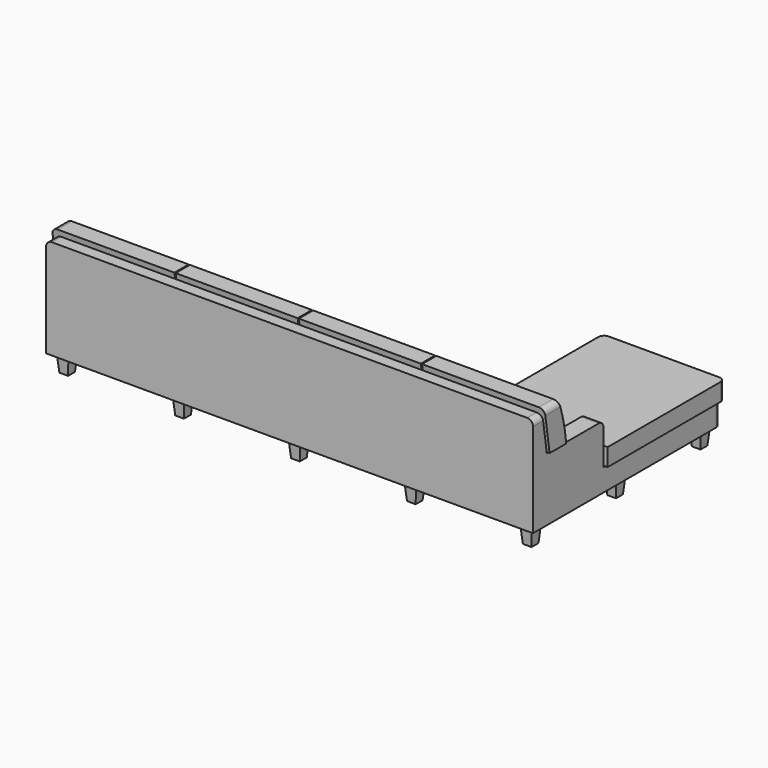
from build123d import *

# Parameters (mm, degrees)
F1_DEPTH       = 4150
F2_W           = 1000
F2_H           = 1100
F3_DEPTH       = 190
F4_W           = 150
F4_H           = 350
F5_DEPTH       = 750
F6_W           = 150
F6_H           = 540
F7_DEPTH       = 750
F9_DEPTH       = 150
F11_DEPTH      = 4175
F11_DEPTH_BACK = 25
F12_W          = 185
F12_H          = 210
F13_DEPTH      = 2020.001
F14_W          = 10
F14_H          = 920
F15_DEPTH      = 560.001
F15_DEPTH_BACK = 340.001
F16_R          = 50
F16_2_R        = 50
F16_3_R        = 50
F17_W          = 100
F17_H          = 100
F18_DEPTH      = 150
F18_TAPER      = 5


with BuildPart() as f1:
    # F0 (on Right) → F1 (new body)
    with BuildSketch(Plane.YZ):
        Polygon((0, 1000), (0, 150), (900, 150), (900, 340), (200, 340), (100, 1000), align=None)
    extrude(amount=F1_DEPTH)

    # F2 (on face) → F3 (join, through all)
    with BuildSketch(Plane(origin=(0, 0, 150), x_dir=(1, 0, 0), z_dir=(0, 0, -1))):
        with Locations((3650, -1450)):
            Rectangle(F2_W, F2_H)
    extrude(amount=-F3_DEPTH)

    # F4 (on Front) → F5 (join)
    with BuildSketch(Plane.XZ):
        with Locations((75, 515)):
            Rectangle(F4_W, F4_H)
    extrude(amount=-F5_DEPTH)

    # F6 (on Front) → F7 (join)
    with BuildSketch(Plane.XZ):
        with Locations((4075, 420)):
            Rectangle(F6_W, F6_H)
    extrude(amount=-F7_DEPTH)

    # F16
    f16_edges = [f1.edges().sort_by_distance(p)[0] for p in [
        (4150, 50, 1000),
        (4075, 750, 690),
        (4150, 2000, 245),
        (3150, 2000, 245),
        (0, 900, 245),
        (75, 750, 690),
        (0, 50, 1000),
    ]]
    fillet(f16_edges, radius=F16_R)


with BuildPart() as f9:
    # F8 (on face) → F9 (new body)
    with BuildSketch(Plane.XY.offset(340)):
        Polygon((3980, 770), (4170, 770), (4170, 2020), (3130, 2020), (3130, 920), (-20, 920), (-20, 770), (170, 770), (170, 220), (3980, 220), align=None)
    extrude(amount=F9_DEPTH)


with BuildPart() as f11:
    # F10 (on Right) → F11 (new body, two sides)
    with BuildSketch(Plane.YZ) as f11_sk:
        with BuildLine():
            Line((244.1362357722, 1050), (92.4242424242, 1050))
            Line((92.4242424242, 1050), (177.2727272727, 490))
            Line((177.2727272727, 490), (328.9847206207, 490))
            ThreePointArc((328.9847206207, 490), (313.2319068561, 774.0411255545), (244.1362357722, 1050))
        make_face()
    extrude(amount=F11_DEPTH)
    extrude(f11_sk.sketch, amount=-F11_DEPTH_BACK)

    # F12 (on Front) → F13 (cut, through all)
    with BuildSketch(Plane.XZ):
        with Locations((4082.5, 595)):
            Rectangle(F12_W, F12_H)
        with Locations((67.5, 595)):
            Rectangle(F12_W, F12_H)
    extrude(amount=-F13_DEPTH, mode=Mode.SUBTRACT)


with BuildPart() as f15_tool:
    # F14 (on face) → F15 (new body, two sides)
    with BuildSketch(Plane.XY.offset(490)) as f15_sk:
        with Locations((3125, 460)):
            Rectangle(F14_W, F14_H)
        with Locations((2075, 460)):
            Rectangle(F14_W, F14_H)
        with Locations((1025, 460)):
            Rectangle(F14_W, F14_H)
    extrude(amount=F15_DEPTH)
    extrude(f15_sk.sketch, amount=-F15_DEPTH_BACK)


with BuildPart() as f9_1:
    add(f9.part)

    # F15: cut by f15_tool
    add(f15_tool.part, mode=Mode.SUBTRACT)

    # F16#2
    f16_2_edges = [f9_1.edges().sort_by_distance(p)[0] for p in [
        (3130, 2020, 415),
        (4170, 2020, 415),
        (-20, 920, 415),
    ]]
    fillet(f16_2_edges, radius=F16_2_R)


with BuildPart() as f11_1:
    add(f11.part)

    # F15: cut by f15_tool
    add(f15_tool.part, mode=Mode.SUBTRACT)

    # F16#3
    f16_3_edges = [f11_1.edges().sort_by_distance(p)[0] for p in [
        (4175, 168.280239, 1050),
        (-25, 168.280239, 1050),
    ]]
    fillet(f16_3_edges, radius=F16_3_R)


with BuildPart() as f18:
    # F17 (on face) → F18 (new body, through all)
    with BuildSketch(Plane(origin=(0, 0, 150), x_dir=(1, 0, 0), z_dir=(0, 0, -1))):
        with Locations((100, -100)):
            Rectangle(F17_W, F17_H)
    extrude(amount=F18_DEPTH, taper=F18_TAPER)


with BuildPart() as f18b:
    # F17 (on face) → F18, piece 2 (new body, through all)
    with BuildSketch(Plane(origin=(0, 0, 150), x_dir=(1, 0, 0), z_dir=(0, 0, -1))):
        with Locations((1087.5, -100)):
            Rectangle(F17_W, F17_H)
    extrude(amount=F18_DEPTH, taper=F18_TAPER)


with BuildPart() as f18c:
    # F17 (on face) → F18, piece 3 (new body, through all)
    with BuildSketch(Plane(origin=(0, 0, 150), x_dir=(1, 0, 0), z_dir=(0, 0, -1))):
        with Locations((2075, -100)):
            Rectangle(F17_W, F17_H)
    extrude(amount=F18_DEPTH, taper=F18_TAPER)


with BuildPart() as f18d:
    # F17 (on face) → F18, piece 4 (new body, through all)
    with BuildSketch(Plane(origin=(0, 0, 150), x_dir=(1, 0, 0), z_dir=(0, 0, -1))):
        with Locations((100, -800)):
            Rectangle(F17_W, F17_H)
    extrude(amount=F18_DEPTH, taper=F18_TAPER)


with BuildPart() as f18e:
    # F17 (on face) → F18, piece 5 (new body, through all)
    with BuildSketch(Plane(origin=(0, 0, 150), x_dir=(1, 0, 0), z_dir=(0, 0, -1))):
        with Locations((1150, -800)):
            Rectangle(F17_W, F17_H)
    extrude(amount=F18_DEPTH, taper=F18_TAPER)


with BuildPart() as f18f:
    # F17 (on face) → F18, piece 6 (new body, through all)
    with BuildSketch(Plane(origin=(0, 0, 150), x_dir=(1, 0, 0), z_dir=(0, 0, -1))):
        with Locations((2200, -800)):
            Rectangle(F17_W, F17_H)
    extrude(amount=F18_DEPTH, taper=F18_TAPER)


with BuildPart() as f18g:
    # F17 (on face) → F18, piece 7 (new body, through all)
    with BuildSketch(Plane(origin=(0, 0, 150), x_dir=(1, 0, 0), z_dir=(0, 0, -1))):
        Polygon((4000, -1850), (4000, -1900), (4000, -1950), (4100, -1950), (4100, -1850), align=None)
    extrude(amount=F18_DEPTH, taper=F18_TAPER)


with BuildPart() as f18h:
    # F17 (on face) → F18, piece 8 (new body, through all)
    with BuildSketch(Plane(origin=(0, 0, 150), x_dir=(1, 0, 0), z_dir=(0, 0, -1))):
        Polygon((3300, -1850), (3200, -1850), (3200, -1950), (3300, -1950), (3300, -1900), align=None)
    extrude(amount=F18_DEPTH, taper=F18_TAPER)


with BuildPart() as f18i:
    # F17 (on face) → F18, piece 9 (new body, through all)
    with BuildSketch(Plane(origin=(0, 0, 150), x_dir=(1, 0, 0), z_dir=(0, 0, -1))):
        with Locations((4050, -100)):
            Rectangle(F17_W, F17_H)
    extrude(amount=F18_DEPTH, taper=F18_TAPER)


with BuildPart() as f18j:
    # F17 (on face) → F18, piece 10 (new body, through all)
    with BuildSketch(Plane(origin=(0, 0, 150), x_dir=(1, 0, 0), z_dir=(0, 0, -1))):
        with Locations((4050, -1000)):
            Rectangle(F17_W, F17_H)
    extrude(amount=F18_DEPTH, taper=F18_TAPER)


with BuildPart() as f18k:
    # F17 (on face) → F18, piece 11 (new body, through all)
    with BuildSketch(Plane(origin=(0, 0, 150), x_dir=(1, 0, 0), z_dir=(0, 0, -1))):
        with Locations((3250, -800)):
            Rectangle(F17_W, F17_H)
    extrude(amount=F18_DEPTH, taper=F18_TAPER)


with BuildPart() as f18l:
    # F17 (on face) → F18, piece 12 (new body, through all)
    with BuildSketch(Plane(origin=(0, 0, 150), x_dir=(1, 0, 0), z_dir=(0, 0, -1))):
        with Locations((3062.5, -100)):
            Rectangle(F17_W, F17_H)
    extrude(amount=F18_DEPTH, taper=F18_TAPER)


solid = Compound([f1.part, f9_1.part, f11_1.part, f18.part, f18b.part, f18c.part, f18d.part, f18e.part, f18f.part, f18g.part, f18h.part, f18i.part, f18j.part, f18k.part, f18l.part])
